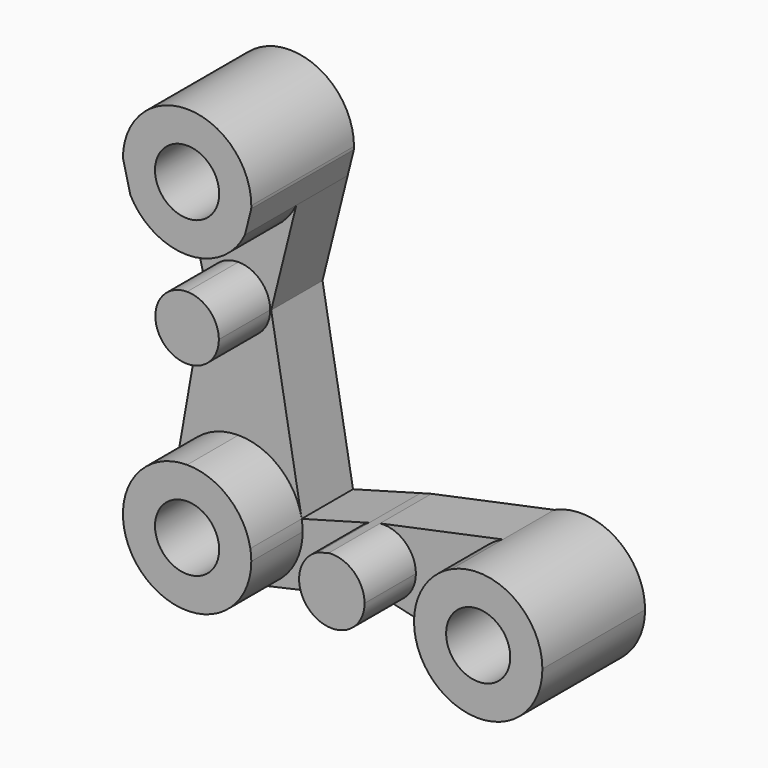
from build123d import *

# Parameters (mm, degrees)
F1_DEPTH = 50.8
F2_DEPTH = 25.4
F3_D     = 25.4
F3_2_D   = 25.4
F3_3_D   = 25.4


# Not quite as in the source:
# - ends of sketch curves that miss each other by under 0.0002 mm in the source are joined


with BuildPart() as f1:
    # F0 (on Front) → F1 (new body)
    with BuildSketch(Plane.XZ):
        with BuildLine():
            ThreePointArc((-115.1953488588, 25.4), (-101.6630890972, 29.30493206), (-92.291660437, 39.8190593902))
            Line((-92.291660437, 39.8190593902), (-89.8185141224, 49.7154453636))
            ThreePointArc((-89.8185141224, 49.7154453636), (-89.8011408351, 50.2575989978), (-89.7953488588, 50.8))
            ThreePointArc((-89.7953488588, 50.8), (-115.0868603739, 76.1997683109), (-140.5944221068, 51.0169749908))
            Line((-140.5944221068, 51.0169749908), (-137.6334657409, 38.8966008725))
            ThreePointArc((-137.6334657409, 38.8966008725), (-128.2875920234, 29.0341283446), (-115.1953488588, 25.4))
        make_face()
    extrude(amount=F1_DEPTH)

    # F3 (through all)
    with Locations(Plane(origin=(0, 0, 0), x_dir=(1, 0, 0), z_dir=(0, 1, 0))):
        with Locations((-115.1953488588, -50.8), (-115.1953488588, 73.1457510495), (0, 73.1457510495)):
            Hole(F3_D / 2)


with BuildPart() as f1b:
    # F0 (on Front) → F1, piece 2 (new body)
    with BuildSketch(Plane.XZ):
        with BuildLine():
            ThreePointArc((-115.1953488588, 12.5662939133), (-127.7616427722, 0), (-115.1953488588, -12.5662939133))
            Line((-115.1953488588, -12.5662939133), (-115.1953488588, 0))
            Line((-115.1953488588, 0), (-115.1953488588, 12.5662939133))
        make_face()
        with BuildLine():
            Line((-115.1953488588, 0), (-115.1953488588, -12.5662939133))
            ThreePointArc((-115.1953488588, -12.5662939133), (-106.3096372183, -8.8857116405), (-102.6290549455, 0))
            ThreePointArc((-102.6290549455, 0), (-106.3096372183, 8.8857116405), (-115.1953488588, 12.5662939133))
            Line((-115.1953488588, 12.5662939133), (-115.1953488588, 0))
        make_face()
    extrude(amount=F1_DEPTH)


with BuildPart() as f1c:
    # F0 (on Front) → F1, piece 3 (new body)
    with BuildSketch(Plane.XZ):
        with BuildLine():
            ThreePointArc((-108.4626208204, -97.6371857392), (-94.9942190368, -88.5429700813), (-89.7953488588, -73.1457510495))
            Line((-89.7953488588, -73.1457510495), (-115.1953488588, -73.1457510495))
            Line((-115.1953488588, -73.1457510495), (-115.1953488588, -47.7457510495))
            ThreePointArc((-115.1953488588, -47.7457510495), (-131.5278604467, -53.6930117763), (-140.212048827, -68.7497616611))
            ThreePointArc((-140.212048827, -68.7497616611), (-132.2891116058, -91.9330679189), (-108.4626208204, -97.6371857392))
        make_face()
        with BuildLine():
            Line((-115.1953488588, -73.1457510495), (-89.7953488588, -73.1457510495))
            ThreePointArc((-89.7953488588, -73.1457510495), (-89.891355303, -70.9394169576), (-90.1786488687, -68.7497617861))
            ThreePointArc((-90.1786488687, -68.7497617861), (-98.8628372224, -53.6930118171), (-115.1953488588, -47.7457510495))
            Line((-115.1953488588, -47.7457510495), (-115.1953488588, -73.1457510495))
        make_face()
    extrude(amount=F1_DEPTH)

    # F3#2 (through all)
    with Locations(Plane(origin=(0, 0, 0), x_dir=(1, 0, 0), z_dir=(0, 1, 0))):
        with Locations((-115.1953488588, -50.8), (-115.1953488588, 73.1457510495), (0, 73.1457510495)):
            Hole(F3_2_D / 2)


with BuildPart() as f1d:
    # F0 (on Front) → F1, piece 4 (new body)
    with BuildSketch(Plane.XZ):
        with BuildLine():
            ThreePointArc((-63.4545843049, -61.4323040872), (-68.8681180563, -66.2110512717), (-70.8812527568, -73.1457510495))
            Line((-70.8812527568, -73.1457510495), (-57.930611074, -73.1457510495))
            Line((-57.930611074, -73.1457510495), (-44.9799693912, -73.1457510495))
            ThreePointArc((-44.9799693912, -73.1457510495), (-49.2128317892, -63.5687241446), (-59.1444326796, -60.2521186247))
            Line((-59.1444326796, -60.2521186247), (-63.4545843049, -61.4323040872))
        make_face()
        with BuildLine():
            Line((-57.930611074, -73.1457510495), (-70.8812527568, -73.1457510495))
            ThreePointArc((-70.8812527568, -73.1457510495), (-66.5244411037, -82.8341567706), (-56.385414216, -86.0038802551))
            ThreePointArc((-56.385414216, -86.0038802551), (-48.2422053529, -81.7395810792), (-44.9799693912, -73.1457510495))
            Line((-44.9799693912, -73.1457510495), (-57.930611074, -73.1457510495))
        make_face()
    extrude(amount=F1_DEPTH)


with BuildPart() as f1e:
    # F0 (on Front) → F1, piece 5 (new body)
    with BuildSketch(Plane.XZ):
        with BuildLine():
            ThreePointArc((-25.4, -73.1457510495), (-21.170469895, -87.1803940597), (-9.8904563446, -96.5410256428))
            ThreePointArc((-9.8904563446, -96.5410256428), (14.0346430102, -94.3162209445), (25.4, -73.1457510495))
            ThreePointArc((25.4, -73.1457510495), (13.7371971399, -51.7810742502), (-10.5408987984, -50.0362410478))
            ThreePointArc((-10.5408987984, -50.0362410478), (-21.3646767993, -59.4085539097), (-25.4, -73.1457510495))
        make_face()
    extrude(amount=F1_DEPTH)

    # F3#3 (through all)
    with Locations(Plane(origin=(0, 0, 0), x_dir=(1, 0, 0), z_dir=(0, 1, 0))):
        with Locations((-115.1953488588, -50.8), (-115.1953488588, 73.1457510495), (0, 73.1457510495)):
            Hole(F3_3_D / 2)


with BuildPart() as f2:
    # F0 (on Front) → F2 (new body)
    with BuildSketch(Plane.XZ):
        with BuildLine():
            ThreePointArc((-140.212048827, -68.7497616611), (-131.5278604467, -53.6930117763), (-115.1953488588, -47.7457510495))
            Line((-115.1953488588, -47.7457510495), (-115.1953488588, -12.5662939133))
            ThreePointArc((-115.1953488588, -12.5662939133), (-127.7616427722, 0), (-115.1953488588, 12.5662939133))
            Line((-115.1953488588, 12.5662939133), (-115.1953488588, 25.4))
            ThreePointArc((-115.1953488588, 25.4), (-128.2875920234, 29.0341283446), (-137.6334657409, 38.8966008725))
            Line((-137.6334657409, 38.8966008725), (-128.1311899166, 0))
            Line((-128.1311899166, 0), (-140.212048827, -68.7497616611))
        make_face()
        with BuildLine():
            ThreePointArc((-115.1953488588, -47.7457510495), (-98.8628372224, -53.6930118171), (-90.1786488687, -68.7497617861))
            Line((-90.1786488687, -68.7497617861), (-102.2426021492, 0))
            Line((-102.2426021492, 0), (-92.291660437, 39.8190593902))
            ThreePointArc((-92.291660437, 39.8190593902), (-101.6630890972, 29.30493206), (-115.1953488588, 25.4))
            Line((-115.1953488588, 25.4), (-115.1953488588, 12.5662939133))
            ThreePointArc((-115.1953488588, 12.5662939133), (-106.3096372183, 8.8857116405), (-102.6290549455, 0))
            ThreePointArc((-102.6290549455, 0), (-106.3096372183, -8.8857116405), (-115.1953488588, -12.5662939133))
            Line((-115.1953488588, -12.5662939133), (-115.1953488588, -47.7457510495))
        make_face()
    extrude(amount=F2_DEPTH)


with BuildPart() as f2b:
    # F0 (on Front) → F2, piece 2 (new body)
    with BuildSketch(Plane.XZ):
        with BuildLine():
            ThreePointArc((-90.1786488687, -68.7497617861), (-89.891355303, -70.9394169576), (-89.7953488588, -73.1457510495))
            Line((-89.7953488588, -73.1457510495), (-70.8812527568, -73.1457510495))
            ThreePointArc((-70.8812527568, -73.1457510495), (-68.8681180563, -66.2110512717), (-63.4545843049, -61.4323040872))
            Line((-63.4545843049, -61.4323040872), (-90.1786488687, -68.7497617861))
        make_face()
        with BuildLine():
            Line((-70.8812527568, -73.1457510495), (-89.7953488588, -73.1457510495))
            ThreePointArc((-89.7953488588, -73.1457510495), (-94.9942190368, -88.5429700813), (-108.4626208204, -97.6371857392))
            Line((-108.4626208204, -97.6371857392), (-56.385414216, -86.0038802551))
            ThreePointArc((-56.385414216, -86.0038802551), (-66.5244411037, -82.8341567706), (-70.8812527568, -73.1457510495))
        make_face()
    extrude(amount=F2_DEPTH)


with BuildPart() as f2c:
    # F0 (on Front) → F2, piece 3 (new body)
    with BuildSketch(Plane.XZ):
        with BuildLine():
            ThreePointArc((-59.1444326796, -60.2521186247), (-49.2128317892, -63.5687241446), (-44.9799693912, -73.1457510495))
            Line((-44.9799693912, -73.1457510495), (-25.4, -73.1457510495))
            ThreePointArc((-25.4, -73.1457510495), (-21.3646767993, -59.4085539097), (-10.5408987984, -50.0362410478))
            Line((-10.5408987984, -50.0362410478), (-59.1444326796, -60.2521186247))
        make_face()
        with BuildLine():
            ThreePointArc((-44.9799693912, -73.1457510495), (-48.2422053529, -81.7395810792), (-56.385414216, -86.0038802551))
            Line((-56.385414216, -86.0038802551), (-9.8904563446, -96.5410256428))
            ThreePointArc((-9.8904563446, -96.5410256428), (-21.170469895, -87.1803940597), (-25.4, -73.1457510495))
            Line((-25.4, -73.1457510495), (-44.9799693912, -73.1457510495))
        make_face()
    extrude(amount=F2_DEPTH)


solid = Compound([f1.part, f1b.part, f1c.part, f1d.part, f1e.part, f2.part, f2b.part, f2c.part])
